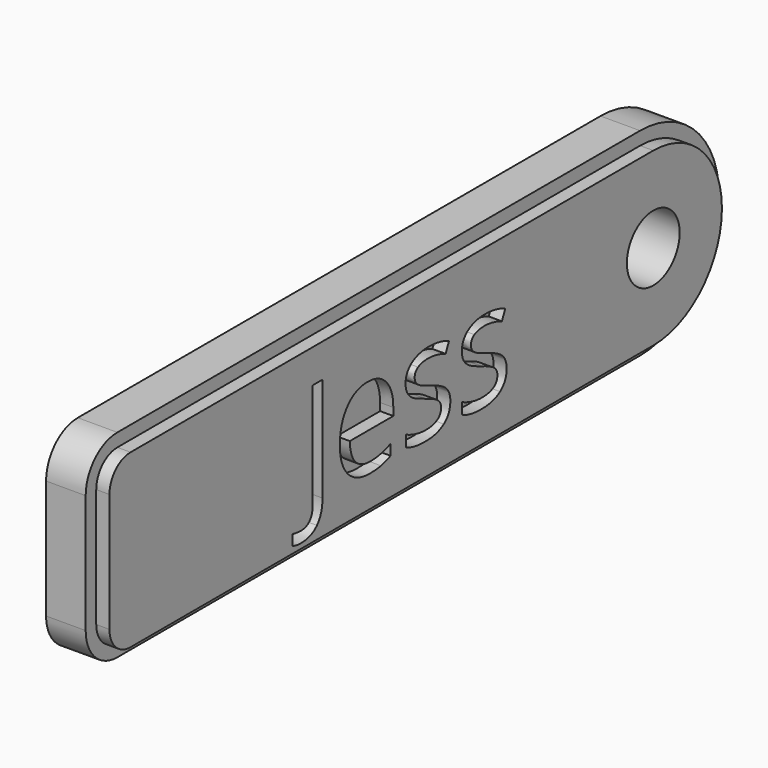
from build123d import *

# Parameters (mm, degrees)
F0_R     = 2.5
F1_DEPTH = 3
F2_R     = 2.5
F3_DEPTH = 1


# Not quite as in the source:
# - a feature names something its author has since deleted; it is built from what else it names


with BuildPart() as f1:
    # F0 (on Right) → F1 (new body)
    with BuildSketch(Plane.YZ):
        with BuildLine():
            Line((22.7894122154, 7.5), (-26.7105877846, 7.5))
            ThreePointArc((-26.7105877846, 7.5), (-28.8319081282, 6.6213203436), (-29.7105877846, 4.5))
            Line((-29.7105877846, 4.5), (-29.7105877846, -4.5))
            ThreePointArc((-29.7105877846, -4.5), (-28.8319081282, -6.6213203436), (-26.7105877846, -7.5))
            Line((-26.7105877846, -7.5), (22.7894122154, -7.5))
            ThreePointArc((22.7894122154, -7.5), (30.2894122154, 0), (22.7894122154, 7.5))
        make_face()
        with Locations((22.7894122154, 0)):
            Circle(F0_R, mode=Mode.SUBTRACT)
    extrude(amount=F1_DEPTH)

    # F2 (on face) → F3 (join)
    with BuildSketch(Plane.YZ.offset(3)):
        with BuildLine():
            Line((22.7894122154, 6.5), (-26.7105877846, 6.5))
            ThreePointArc((-26.7105877846, 6.5), (-28.124801347, 5.9142135624), (-28.7105877846, 4.5))
            Line((-28.7105877846, 4.5), (-28.7105877846, -4.5))
            ThreePointArc((-28.7105877846, -4.5), (-28.124801347, -5.9142135624), (-26.7105877846, -6.5))
            Line((-26.7105877846, -6.5), (22.7894122154, -6.5))
            ThreePointArc((22.7894122154, -6.5), (29.2894122154, 0), (22.7894122154, 6.5))
        make_face()
        with BuildLine():
            add(Edge.make_bspline(
                [(-9.0594911449, -5.5533798952), (-9.5833125468, -6.1234721876), (-10.5663507109, -6.1234721876)],
                knots=[0, 0, 0, 1, 1, 1], degree=2))
            add(Edge.make_bspline(
                [(-10.5663507109, -6.1234721876), (-11.0779496134, -6.1234721876), (-11.3730356697, -5.9768021951)],
                knots=[0, 0, 0, 1, 1, 1], degree=2))
            Line((-11.3730356697, -5.9768021951), (-11.3730356697, -5.1858318783))
            add(Edge.make_bspline(
                [(-11.3730356697, -5.1858318783), (-10.9854078324, -5.2940883013), (-10.5663507109, -5.2940883013)],
                knots=[0, 0, 0, 1, 1, 1], degree=2))
            add(Edge.make_bspline(
                [(-10.5663507109, -5.2940883013), (-10.0250685957, -5.2940883013), (-9.74395111, -4.9666999252)],
                knots=[0, 0, 0, 1, 1, 1], degree=2))
            add(Edge.make_bspline(
                [(-9.74395111, -4.9666999252), (-9.4628336243, -4.639311549), (-9.4628336243, -4.0229483662)],
                knots=[0, 0, 0, 1, 1, 1], degree=2))
            Line((-9.4628336243, -4.0229483662), (-9.4628336243, 3.9548515839))
            Line((-9.4628336243, 3.9548515839), (-8.5356697431, 3.9548515839))
            Line((-8.5356697431, 3.9548515839), (-8.5356697431, -3.9461212272))
            add(Edge.make_bspline(
                [(-8.5356697431, -3.9461212272), (-8.5356697431, -4.9832876029), (-9.0594911449, -5.5533798952)],
                knots=[0, 0, 0, 1, 1, 1], degree=2))
        make_face(mode=Mode.SUBTRACT)
        with BuildLine():
            add(Edge.make_bspline(
                [(-2.9953853829, -4.0421551509), (-3.4231728611, -4.1329508606), (-4.0290596159, -4.1329508606)],
                knots=[0, 0, 0, 1, 1, 1], degree=2))
            add(Edge.make_bspline(
                [(-4.0290596159, -4.1329508606), (-5.3543277625, -4.1329508606), (-6.1217261162, -3.3245198304)],
                knots=[0, 0, 0, 1, 1, 1], degree=2))
            add(Edge.make_bspline(
                [(-6.1217261162, -3.3245198304), (-6.8891244699, -2.5160888002), (-6.8891244699, -1.0825642305)],
                knots=[0, 0, 0, 1, 1, 1], degree=2))
            add(Edge.make_bspline(
                [(-6.8891244699, -1.0825642305), (-6.8891244699, 0.36492891), (-6.1767273634, 1.216138688)],
                knots=[0, 0, 0, 1, 1, 1], degree=2))
            add(Edge.make_bspline(
                [(-6.1767273634, 1.216138688), (-5.4643302569, 2.067348466), (-4.2630331754, 2.067348466)],
                knots=[0, 0, 0, 1, 1, 1], degree=2))
            add(Edge.make_bspline(
                [(-4.2630331754, 2.067348466), (-3.1403093041, 2.067348466), (-2.4855325518, 1.3278872537)],
                knots=[0, 0, 0, 1, 1, 1], degree=2))
            add(Edge.make_bspline(
                [(-2.4855325518, 1.3278872537), (-1.8307557995, 0.5884260414), (-1.8307557995, -0.6233474682)],
                knots=[0, 0, 0, 1, 1, 1], degree=2))
            Line((-1.8307557995, -0.6233474682), (-1.8307557995, -1.1960588675))
            Line((-1.8307557995, -1.1960588675), (-5.9497380893, -1.1960588675))
            add(Edge.make_bspline(
                [(-5.9497380893, -1.1960588675), (-5.9218009479, -2.2489398853), (-5.4171863308, -2.7945871788)],
                knots=[0, 0, 0, 1, 1, 1], degree=2))
            add(Edge.make_bspline(
                [(-5.4171863308, -2.7945871788), (-4.9125717136, -3.3402344724), (-3.9958842604, -3.3402344724)],
                knots=[0, 0, 0, 1, 1, 1], degree=2))
            add(Edge.make_bspline(
                [(-3.9958842604, -3.3402344724), (-3.0303068097, -3.3402344724), (-2.0874282864, -2.936891993)],
                knots=[0, 0, 0, 1, 1, 1], degree=2))
            Line((-2.0874282864, -2.936891993), (-2.0874282864, -3.7453230232))
            add(Edge.make_bspline(
                [(-2.0874282864, -3.7453230232), (-2.5675979047, -3.9513594413), (-2.9953853829, -4.0421551509)],
                knots=[0, 0, 0, 1, 1, 1], degree=2))
        make_face(mode=Mode.SUBTRACT)
        with BuildLine():
            add(Edge.make_bspline(
                [(3.1979296583, -1.4038413569), (3.5715889249, -1.7967074083), (3.5715889249, -2.3921177351)],
                knots=[0, 0, 0, 1, 1, 1], degree=2))
            add(Edge.make_bspline(
                [(3.5715889249, -2.3921177351), (3.5715889249, -3.2267398354), (2.9499875281, -3.679845348)],
                knots=[0, 0, 0, 1, 1, 1], degree=2))
            add(Edge.make_bspline(
                [(2.9499875281, -3.679845348), (2.3283861312, -4.1329508606), (1.2039161886, -4.1329508606)],
                knots=[0, 0, 0, 1, 1, 1], degree=2))
            add(Edge.make_bspline(
                [(1.2039161886, -4.1329508606), (0.0148416064, -4.1329508606), (-0.650411574, -3.7557994512)],
                knots=[0, 0, 0, 1, 1, 1], degree=2))
            Line((-0.650411574, -3.7557994512), (-0.650411574, -2.9159391369))
            add(Edge.make_bspline(
                [(-0.650411574, -2.9159391369), (-0.2191319531, -3.1341980544), (0.2741332003, -3.2590421552)],
                knots=[0, 0, 0, 1, 1, 1], degree=2))
            add(Edge.make_bspline(
                [(0.2741332003, -3.2590421552), (0.7673983537, -3.3838862559), (1.226615116, -3.3838862559)],
                knots=[0, 0, 0, 1, 1, 1], degree=2))
            add(Edge.make_bspline(
                [(1.226615116, -3.3838862559), (1.9355200798, -3.3838862559), (2.3170366675, -3.1577700175)],
                knots=[0, 0, 0, 1, 1, 1], degree=2))
            add(Edge.make_bspline(
                [(2.3170366675, -3.1577700175), (2.6985532552, -2.931653779), (2.6985532552, -2.4671988027)],
                knots=[0, 0, 0, 1, 1, 1], degree=2))
            add(Edge.make_bspline(
                [(2.6985532552, -2.4671988027), (2.6985532552, -2.1179845348), (2.3964829134, -1.8700424046)],
                knots=[0, 0, 0, 1, 1, 1], degree=2))
            add(Edge.make_bspline(
                [(2.3964829134, -1.8700424046), (2.0944125717, -1.6221002744), (1.2143926166, -1.2833624345)],
                knots=[0, 0, 0, 1, 1, 1], degree=2))
            add(Edge.make_bspline(
                [(1.2143926166, -1.2833624345), (0.3797705163, -0.9725617361), (0.0279371414, -0.7403342479)],
                knots=[0, 0, 0, 1, 1, 1], degree=2))
            add(Edge.make_bspline(
                [(0.0279371414, -0.7403342479), (-0.3238962335, -0.5081067598), (-0.4958842604, -0.2138937391)],
                knots=[0, 0, 0, 1, 1, 1], degree=2))
            add(Edge.make_bspline(
                [(-0.4958842604, -0.2138937391), (-0.6678722874, 0.0803192816), (-0.6678722874, 0.4888999751)],
                knots=[0, 0, 0, 1, 1, 1], degree=2))
            add(Edge.make_bspline(
                [(-0.6678722874, 0.4888999751), (-0.6678722874, 1.2205038663), (-0.0724619606, 1.6439261661)],
                knots=[0, 0, 0, 1, 1, 1], degree=2))
            add(Edge.make_bspline(
                [(-0.0724619606, 1.6439261661), (0.5229483662, 2.067348466), (1.5583686705, 2.067348466)],
                knots=[0, 0, 0, 1, 1, 1], degree=2))
            add(Edge.make_bspline(
                [(1.5583686705, 2.067348466), (2.5239461212, 2.067348466), (3.4476178598, 1.6744824146)],
                knots=[0, 0, 0, 1, 1, 1], degree=2))
            Line((3.4476178598, 1.6744824146), (3.124594662, 0.9376403093))
            add(Edge.make_bspline(
                [(3.124594662, 0.9376403093), (2.2253679222, 1.3078074333), (1.4937640309, 1.3078074333)],
                knots=[0, 0, 0, 1, 1, 1], degree=2))
            add(Edge.make_bspline(
                [(1.4937640309, 1.3078074333), (0.8494637067, 1.3078074333), (0.5220753305, 1.1061361936)],
                knots=[0, 0, 0, 1, 1, 1], degree=2))
            add(Edge.make_bspline(
                [(0.5220753305, 1.1061361936), (0.1946869544, 0.9044649539), (0.1946869544, 0.5500124719)],
                knots=[0, 0, 0, 1, 1, 1], degree=2))
            add(Edge.make_bspline(
                [(0.1946869544, 0.5500124719), (0.1946869544, 0.3090546271), (0.3177849838, 0.1405587428)],
                knots=[0, 0, 0, 1, 1, 1], degree=2))
            add(Edge.make_bspline(
                [(0.3177849838, 0.1405587428), (0.4408830132, -0.0279371414), (0.7132701422, -0.1807183836)],
                knots=[0, 0, 0, 1, 1, 1], degree=2))
            add(Edge.make_bspline(
                [(0.7132701422, -0.1807183836), (0.9856572711, -0.3334996258), (1.7609129459, -0.6233474682)],
                knots=[0, 0, 0, 1, 1, 1], degree=2))
            add(Edge.make_bspline(
                [(1.7609129459, -0.6233474682), (2.8242703916, -1.0109753056), (3.1979296583, -1.4038413569)],
                knots=[0, 0, 0, 1, 1, 1], degree=2))
        make_face(mode=Mode.SUBTRACT)
        with BuildLine():
            add(Edge.make_bspline(
                [(8.5286854577, -1.4038413569), (8.9023447244, -1.7967074083), (8.9023447244, -2.3921177351)],
                knots=[0, 0, 0, 1, 1, 1], degree=2))
            add(Edge.make_bspline(
                [(8.9023447244, -2.3921177351), (8.9023447244, -3.2267398354), (8.2807433275, -3.679845348)],
                knots=[0, 0, 0, 1, 1, 1], degree=2))
            add(Edge.make_bspline(
                [(8.2807433275, -3.679845348), (7.6591419307, -4.1329508606), (6.534671988, -4.1329508606)],
                knots=[0, 0, 0, 1, 1, 1], degree=2))
            add(Edge.make_bspline(
                [(6.534671988, -4.1329508606), (5.3455974058, -4.1329508606), (4.6803442255, -3.7557994512)],
                knots=[0, 0, 0, 1, 1, 1], degree=2))
            Line((4.6803442255, -3.7557994512), (4.6803442255, -2.9159391369))
            add(Edge.make_bspline(
                [(4.6803442255, -2.9159391369), (5.1116238463, -3.1341980544), (5.6048889998, -3.2590421552)],
                knots=[0, 0, 0, 1, 1, 1], degree=2))
            add(Edge.make_bspline(
                [(5.6048889998, -3.2590421552), (6.0981541532, -3.3838862559), (6.5573709154, -3.3838862559)],
                knots=[0, 0, 0, 1, 1, 1], degree=2))
            add(Edge.make_bspline(
                [(6.5573709154, -3.3838862559), (7.2662758793, -3.3838862559), (7.6477924669, -3.1577700175)],
                knots=[0, 0, 0, 1, 1, 1], degree=2))
            add(Edge.make_bspline(
                [(7.6477924669, -3.1577700175), (8.0293090546, -2.931653779), (8.0293090546, -2.4671988027)],
                knots=[0, 0, 0, 1, 1, 1], degree=2))
            add(Edge.make_bspline(
                [(8.0293090546, -2.4671988027), (8.0293090546, -2.1179845348), (7.7272387129, -1.8700424046)],
                knots=[0, 0, 0, 1, 1, 1], degree=2))
            add(Edge.make_bspline(
                [(7.7272387129, -1.8700424046), (7.4251683712, -1.6221002744), (6.5451484161, -1.2833624345)],
                knots=[0, 0, 0, 1, 1, 1], degree=2))
            add(Edge.make_bspline(
                [(6.5451484161, -1.2833624345), (5.7105263158, -0.9725617361), (5.3586929409, -0.7403342479)],
                knots=[0, 0, 0, 1, 1, 1], degree=2))
            add(Edge.make_bspline(
                [(5.3586929409, -0.7403342479), (5.006859566, -0.5081067598), (4.834871539, -0.2138937391)],
                knots=[0, 0, 0, 1, 1, 1], degree=2))
            add(Edge.make_bspline(
                [(4.834871539, -0.2138937391), (4.6628835121, 0.0803192816), (4.6628835121, 0.4888999751)],
                knots=[0, 0, 0, 1, 1, 1], degree=2))
            add(Edge.make_bspline(
                [(4.6628835121, 0.4888999751), (4.6628835121, 1.2205038663), (5.2582938389, 1.6439261661)],
                knots=[0, 0, 0, 1, 1, 1], degree=2))
            add(Edge.make_bspline(
                [(5.2582938389, 1.6439261661), (5.8537041656, 2.067348466), (6.8891244699, 2.067348466)],
                knots=[0, 0, 0, 1, 1, 1], degree=2))
            add(Edge.make_bspline(
                [(6.8891244699, 2.067348466), (7.8547019207, 2.067348466), (8.7783736593, 1.6744824146)],
                knots=[0, 0, 0, 1, 1, 1], degree=2))
            Line((8.7783736593, 1.6744824146), (8.4553504615, 0.9376403093))
            add(Edge.make_bspline(
                [(8.4553504615, 0.9376403093), (7.5561237216, 1.3078074333), (6.8245198304, 1.3078074333)],
                knots=[0, 0, 0, 1, 1, 1], degree=2))
            add(Edge.make_bspline(
                [(6.8245198304, 1.3078074333), (6.1802195061, 1.3078074333), (5.85283113, 1.1061361936)],
                knots=[0, 0, 0, 1, 1, 1], degree=2))
            add(Edge.make_bspline(
                [(5.85283113, 1.1061361936), (5.5254427538, 0.9044649539), (5.5254427538, 0.5500124719)],
                knots=[0, 0, 0, 1, 1, 1], degree=2))
            add(Edge.make_bspline(
                [(5.5254427538, 0.5500124719), (5.5254427538, 0.3090546271), (5.6485407832, 0.1405587428)],
                knots=[0, 0, 0, 1, 1, 1], degree=2))
            add(Edge.make_bspline(
                [(5.6485407832, 0.1405587428), (5.7716388127, -0.0279371414), (6.0440259416, -0.1807183836)],
                knots=[0, 0, 0, 1, 1, 1], degree=2))
            add(Edge.make_bspline(
                [(6.0440259416, -0.1807183836), (6.3164130706, -0.3334996258), (7.0916687453, -0.6233474682)],
                knots=[0, 0, 0, 1, 1, 1], degree=2))
            add(Edge.make_bspline(
                [(7.0916687453, -0.6233474682), (8.1550261911, -1.0109753056), (8.5286854577, -1.4038413569)],
                knots=[0, 0, 0, 1, 1, 1], degree=2))
        make_face(mode=Mode.SUBTRACT)
        with Locations((22.7894122154, 0)):
            Circle(F2_R, mode=Mode.SUBTRACT)
    extrude(amount=F3_DEPTH)


solid = f1.part
